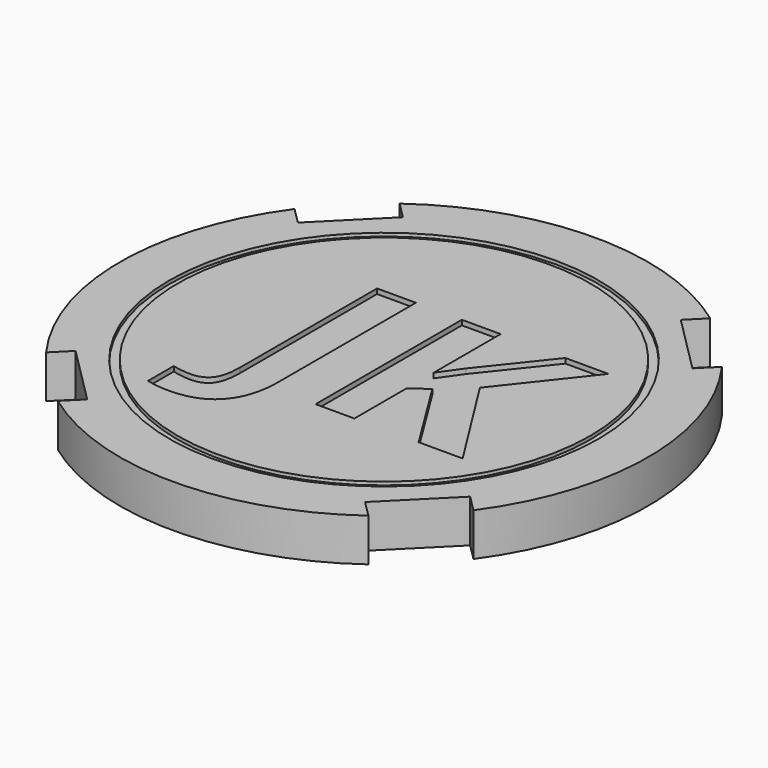
from build123d import *

# Parameters (mm, degrees)
F0_R          = 20.32
F1_DEPTH      = 3.302
F6_DEPTH      = 3.302
F7_R          = 16.51
F7_R_2        = 15.875
F8_DEPTH      = 0.254
F2_TEXT_SIZE  = 8.7192824304
F9_DEPTH      = 0.381
F3_TEXT_SIZE  = 8.8355448193
F10_DEPTH     = 0.381
F4_TEXT_SIZE  = 6.4111328842
F11_DEPTH     = 0.381
F12_TEXT_SIZE = 19.6993015272
F13_DEPTH     = 0.381


# Not quite as in the source:
# - Text() gives the source's letters only with a copy of the font that has no kerning and outlines rounded to 1/6400 em; it was checked with that copy


with BuildPart() as f1:
    # F0 (on Top) → F1 (new body)
    with BuildSketch(Plane.XY):
        Circle(F0_R)
    extrude(amount=F1_DEPTH)

    # F5 (on face) → F6 (cut)
    with BuildSketch(Plane(origin=(0, 0, 0), x_dir=(1, 0, 0), z_dir=(0, 0, -1))):
        with BuildLine():
            Line((-16.4369943958, 11.9468663353), (-15.1766328446, 10.6865047841))
            Line((-15.1766328446, 10.6865047841), (-10.6865047841, 15.1766328446))
            Line((-10.6865047841, 15.1766328446), (-11.9468663353, 16.4369943958))
            ThreePointArc((-11.9468663353, 16.4369943958), (-14.3684097937, 14.3684097937), (-16.4369943958, 11.9468663353))
        make_face()
        with BuildLine():
            Line((-10.6865047841, -15.1766328446), (-15.1766328446, -10.6865047841))
            Line((-15.1766328446, -10.6865047841), (-16.4369943958, -11.9468663353))
            ThreePointArc((-16.4369943958, -11.9468663353), (-14.3684097937, -14.3684097937), (-11.9468663353, -16.4369943958))
            Line((-11.9468663353, -16.4369943958), (-10.6865047841, -15.1766328446))
        make_face()
        with BuildLine():
            Line((15.1766328446, -10.6865047841), (10.6865047841, -15.1766328446))
            Line((10.6865047841, -15.1766328446), (11.9468663353, -16.4369943958))
            ThreePointArc((11.9468663353, -16.4369943958), (14.3684097937, -14.3684097937), (16.4369943958, -11.9468663353))
            Line((16.4369943958, -11.9468663353), (15.1766328446, -10.6865047841))
        make_face()
        with BuildLine():
            Line((10.6865047841, 15.1766328446), (15.1766328446, 10.6865047841))
            Line((15.1766328446, 10.6865047841), (16.4369943958, 11.9468663353))
            ThreePointArc((16.4369943958, 11.9468663353), (14.3684097937, 14.3684097937), (11.9468663353, 16.4369943958))
            Line((11.9468663353, 16.4369943958), (10.6865047841, 15.1766328446))
        make_face()
    extrude(amount=-F6_DEPTH, mode=Mode.SUBTRACT)

    # F7 (on face) → F8 (cut)
    with BuildSketch(Plane.XY.offset(3.302)):
        Circle(F7_R)
        Circle(F7_R_2, mode=Mode.SUBTRACT)
    extrude(amount=-F8_DEPTH, mode=Mode.SUBTRACT)

    # F2 (on face) → F9 (cut)
    with BuildSketch(Plane(origin=(0, 0, 0), x_dir=(1, 0, 0), z_dir=(0, 0, -1))):
        with Locations((-19.4460434017, -3.138941675)):
            Text('Bachelor', F2_TEXT_SIZE, font='Open Sans', font_style=FontStyle.BOLD, text_align=(TextAlign.LEFT, TextAlign.BOTTOM))
    extrude(amount=-F9_DEPTH, mode=Mode.SUBTRACT)

    # F3 (on face) → F10 (cut)
    with BuildSketch(Plane(origin=(0, 0, 0), x_dir=(1, 0, 0), z_dir=(0, 0, -1))):
        with Locations((-8.001, 8.218941675)):
            Text("AJ's", F3_TEXT_SIZE, font='Open Sans', font_style=FontStyle.BOLD, text_align=(TextAlign.LEFT, TextAlign.BOTTOM))
    extrude(amount=-F10_DEPTH, mode=Mode.SUBTRACT)

    # F4 (on face) → F11 (cut)
    with BuildSketch(Plane(origin=(0, 0, 0), x_dir=(1, 0, 0), z_dir=(0, 0, -1))):
        with Locations((-8.8278294597, -12.8349573516)):
            Text('Party', F4_TEXT_SIZE, font='Open Sans', font_style=FontStyle.BOLD, text_align=(TextAlign.LEFT, TextAlign.BOTTOM))
    extrude(amount=-F11_DEPTH, mode=Mode.SUBTRACT)

    # F12 (on face) → F13 (cut)
    with BuildSketch(Plane.XY.offset(3.302)):
        with Locations((-7.8812596188, -7.0917485498)):
            Text('JK', F12_TEXT_SIZE, font='Open Sans', font_style=FontStyle.BOLD, text_align=(TextAlign.LEFT, TextAlign.BOTTOM))
    extrude(amount=-F13_DEPTH, mode=Mode.SUBTRACT)


solid = f1.part
